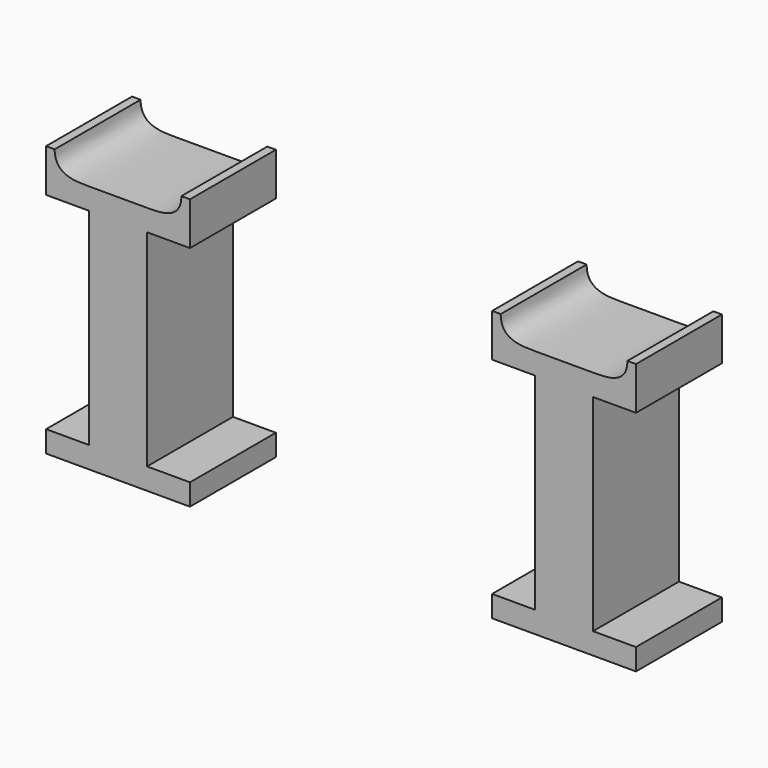
from build123d import *

# Parameters (mm, degrees)
F0_W     = 13.5
F0_H     = 48
F0_H_2   = 5
F0_W_2   = 10
F1_DEPTH = 25
F2_DEPTH = 207


# Not quite as in the source:
# - an extrude ends at something that could not be found from the text; its depth is read off the source's solid


with BuildPart() as f1:
    # F0 (on Front) → F1 (new body)
    with BuildSketch(Plane.XZ):
        with BuildLine():
            Line((-67.1541336304, 32.7363717356), (-69.1541336304, 32.7363717356))
            Line((-69.1541336304, 32.7363717356), (-69.1541336304, 22.7363717356))
            Line((-69.1541336304, 22.7363717356), (-59.1541336304, 22.7363717356))
            Line((-59.1541336304, 22.7363717356), (-45.6541336304, 22.7363717356))
            Line((-45.6541336304, 22.7363717356), (-35.6541336304, 22.7363717356))
            Line((-35.6541336304, 22.7363717356), (-35.6541336304, 32.7363717356))
            Line((-35.6541336304, 32.7363717356), (-37.6541336304, 32.7363717356))
            add(Edge.make_bspline(
                [(-67.1541336304, 32.7363717356), (-67.1541336304, 27.7363717356), (-58.6117428449, 27.7363717356), (-52.4038602705, 27.7363717356), (-46.2003270582, 27.7363717356), (-37.6541336304, 27.7363717356), (-37.6541336304, 32.7363717356)],
                knots=[0, 0, 0, 0, 0.2708316482, 0.5000076733, 0.7291293946, 1, 1, 1, 1], degree=3))
        make_face()
        with BuildLine():
            Line((-37.6541336304, 32.7363717356), (-67.1541336304, 32.7363717356))
            add(Edge.make_bspline(
                [(-67.1541336304, 32.7363717356), (-67.1541336304, 27.7363717356), (-58.6117428449, 27.7363717356), (-52.4038602705, 27.7363717356), (-46.2003270582, 27.7363717356), (-37.6541336304, 27.7363717356), (-37.6541336304, 32.7363717356)],
                knots=[0, 0, 0, 0, 0.2708316482, 0.5000076733, 0.7291293946, 1, 1, 1, 1], degree=3))
        make_face()
        with Locations((-52.4041336304, -1.2636282644)):
            Rectangle(F0_W, F0_H)
        with Locations((-52.4041336304, -27.7636282644)):
            Rectangle(F0_W, F0_H_2)
        with Locations((-64.1541336304, -27.7636282644)):
            Rectangle(F0_W_2, F0_H_2)
        with Locations((-40.6541336304, -27.7636282644)):
            Rectangle(F0_W_2, F0_H_2)
    extrude(amount=F1_DEPTH)


with BuildPart() as f1b:
    # F0 (on Front) → F1, piece 2 (new body)
    with BuildSketch(Plane.XZ):
        with BuildLine():
            Line((36.6787728249, 32.7363717356), (34.6787728249, 32.7363717356))
            Line((34.6787728249, 32.7363717356), (34.6787728249, 22.7363717356))
            Line((34.6787728249, 22.7363717356), (44.6723728249, 22.7363717356))
            Line((44.6723728249, 22.7363717356), (58.1723728249, 22.7363717356))
            Line((58.1723728249, 22.7363717356), (68.1787728249, 22.7363717356))
            Line((68.1787728249, 22.7363717356), (68.1787728249, 32.7363717356))
            Line((68.1787728249, 32.7363717356), (66.1787728249, 32.7363717356))
            add(Edge.make_bspline(
                [(36.6787728249, 32.7363717356), (36.6787728249, 27.7363717356), (45.2171089647, 27.7363717356), (51.4298659754, 27.7363717356), (57.6252269118, 27.7363717356), (66.1787728249, 27.7363717356), (66.1787728249, 32.7363717356)],
                knots=[0, 0, 0, 0, 0.2707968607, 0.5000307078, 0.7290473102, 1, 1, 1, 1], degree=3))
        make_face()
        with BuildLine():
            Line((66.1787728249, 32.7363717356), (36.6787728249, 32.7363717356))
            add(Edge.make_bspline(
                [(36.6787728249, 32.7363717356), (36.6787728249, 27.7363717356), (45.2171089647, 27.7363717356), (51.4298659754, 27.7363717356), (57.6252269118, 27.7363717356), (66.1787728249, 27.7363717356), (66.1787728249, 32.7363717356)],
                knots=[0, 0, 0, 0, 0.2707968607, 0.5000307078, 0.7290473102, 1, 1, 1, 1], degree=3))
        make_face()
        with Locations((51.4223728249, -1.2636282644)):
            Rectangle(F0_W, F0_H)
        with Locations((51.4223728249, -27.7636282644)):
            Rectangle(F0_W, F0_H_2)
        with Locations((39.6723728249, -27.7636282644)):
            Rectangle(F0_W_2, F0_H_2)
        with Locations((63.1723728249, -27.7636282644)):
            Rectangle(F0_W_2, F0_H_2)
    extrude(amount=F1_DEPTH)


with BuildPart() as f2_tool:
    # F1_face (on face) + F0 (on Front) → F2 (new body, through all)
    with BuildSketch(Plane(origin=(-52.4041336304, -25, 3.3224212792), x_dir=(1, 0, 0), z_dir=(0, -1, 0))):
        Polygon((16.75, 29.4139504563), (-16.75, 29.4139504563), (-16.75, 19.4139504563), (-6.75, 19.4139504563), (-6.75, -28.5860495437), (-16.75, -28.5860495437), (-16.75, -33.5860495437), (16.75, -33.5860495437), (16.75, -28.5860495437), (6.75, -28.5860495437), (6.75, 19.4139504563), (16.75, 19.4139504563), align=None)
    with BuildSketch(Plane.XZ):
        with BuildLine():
            Line((66.1787728249, 32.7363717356), (36.6787728249, 32.7363717356))
            add(Edge.make_bspline(
                [(36.6787728249, 32.7363717356), (36.6787728249, 27.7363717356), (45.2171089647, 27.7363717356), (51.4298659754, 27.7363717356), (57.6252269118, 27.7363717356), (66.1787728249, 27.7363717356), (66.1787728249, 32.7363717356)],
                knots=[0, 0, 0, 0, 0.2707968607, 0.5000307078, 0.7290473102, 1, 1, 1, 1], degree=3))
        make_face()
        with BuildLine():
            Line((-37.6541336304, 32.7363717356), (-67.1541336304, 32.7363717356))
            add(Edge.make_bspline(
                [(-67.1541336304, 32.7363717356), (-67.1541336304, 27.7363717356), (-58.6117428449, 27.7363717356), (-52.4038602705, 27.7363717356), (-46.2003270582, 27.7363717356), (-37.6541336304, 27.7363717356), (-37.6541336304, 32.7363717356)],
                knots=[0, 0, 0, 0, 0.2708316482, 0.5000076733, 0.7291293946, 1, 1, 1, 1], degree=3))
        make_face()
    extrude(amount=F2_DEPTH)


with BuildPart() as f1_1:
    add(f1.part)

    # F2: cut by f2_tool
    add(f2_tool.part, mode=Mode.SUBTRACT)


with BuildPart() as f1b_1:
    add(f1b.part)

    # F2: cut by f2_tool
    add(f2_tool.part, mode=Mode.SUBTRACT)


solid = Compound([f1_1.part, f1b_1.part])
